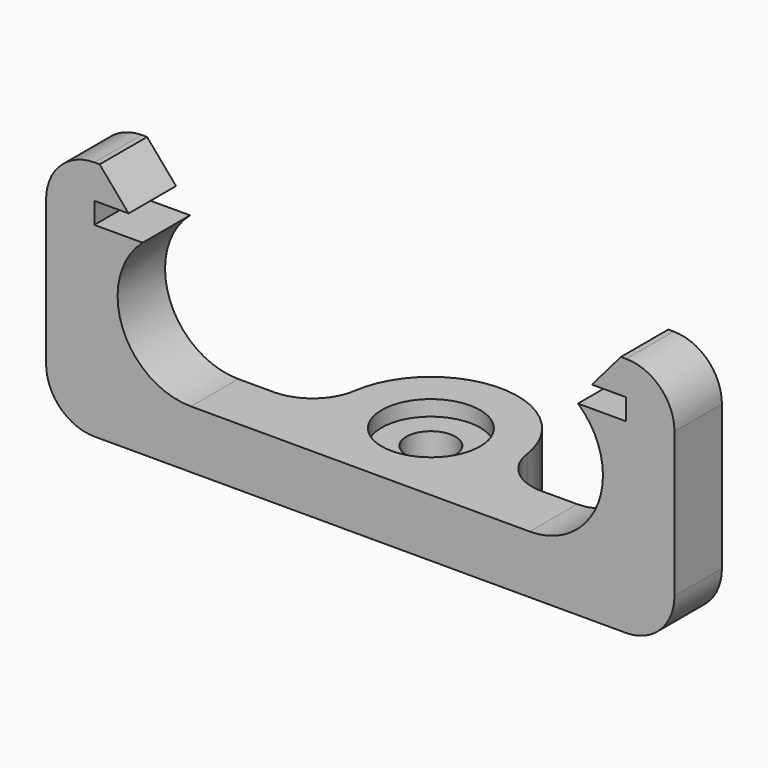
from build123d import *

# Parameters (mm, degrees)
F1_DEPTH = 6
F0_W     = 10
F0_H     = 6.1438416846
F2_DEPTH = 25
F3_DEPTH = 6
F0_R     = 2.55
F4_DEPTH = 4.4
F5_R     = 5
F7_DEPTH = 10


with BuildPart() as f1:
    # F0 (on Top) → F1 (new body)
    with BuildSketch(Plane.XY):
        with BuildLine():
            ThreePointArc((8.4852813742, -3), (0, -9), (-8.4852813742, -3))
            Line((-8.4852813742, -3), (-22.55, -3))
            Line((-22.55, -3), (-22.55, -9.1438416846))
            Line((-22.55, -9.1438416846), (22.55, -9.1438416846))
            Line((22.55, -9.1438416846), (22.55, -3))
            Line((22.55, -3), (8.4852813742, -3))
        make_face()
    extrude(amount=F1_DEPTH)

    # F0 (on Top) → F2 (join)
    with BuildSketch(Plane.XY):
        with Locations((-27.55, -6.0719208423)):
            Rectangle(F0_W, F0_H)
        with Locations((27.55, -6.0719208423)):
            Rectangle(F0_W, F0_H)
    extrude(amount=F2_DEPTH)

    # F0 (on Top) → F3 (join)
    with BuildSketch(Plane.XY):
        with BuildLine():
            ThreePointArc((-4.1243181255, -3), (-1.5773359756, 4.84994961), (5.1, 0))
            ThreePointArc((5.1, 0), (4.84994961, -1.5773359756), (4.1243181255, -3))
            Line((4.1243181255, -3), (8.4852813742, -3))
            ThreePointArc((8.4852813742, -3), (8.8703870369, -1.5219178085), (9, 0))
            ThreePointArc((9, 0), (-1.5219178085, 8.8703870369), (-8.4852813742, -3))
            Line((-8.4852813742, -3), (-4.1243181255, -3))
        make_face()
        with BuildLine():
            ThreePointArc((4.1243181255, -3), (0, -5.1), (-4.1243181255, -3))
            Line((-4.1243181255, -3), (-8.4852813742, -3))
            ThreePointArc((-8.4852813742, -3), (0, -9), (8.4852813742, -3))
            Line((8.4852813742, -3), (4.1243181255, -3))
        make_face()
    extrude(amount=F3_DEPTH)

    # F0 (on Top) → F4 (join)
    with BuildSketch(Plane.XY):
        with BuildLine():
            ThreePointArc((4.1243181255, -3), (4.84994961, -1.5773359756), (5.1, 0))
            ThreePointArc((5.1, 0), (-1.5773359756, 4.84994961), (-4.1243181255, -3))
            Line((-4.1243181255, -3), (4.1243181255, -3))
        make_face()
        Circle(F0_R, mode=Mode.SUBTRACT)
        with BuildLine():
            Line((4.1243181255, -3), (-4.1243181255, -3))
            ThreePointArc((-4.1243181255, -3), (0, -5.1), (4.1243181255, -3))
        make_face()
    extrude(amount=F4_DEPTH)

    # F5
    f5_edges = [f1.edges().sort_by_distance(p)[0] for p in [
        (-8.485281, -3, 3),
        (8.485281, -3, 3),
        (22.55, -6.071921, 6),
        (-22.55, -6.071921, 6),
        (-32.55, -6.071921, 0),
        (32.55, -6.071921, 0),
        (32.55, -6.071921, 25),
        (-32.55, -6.071921, 25),
    ]]
    fillet(f5_edges, radius=F5_R)

    # F6 (on face) → F7 (cut)
    with BuildSketch(Plane.XZ.offset(9.1438416846)):
        Polygon((17.55, 19.3), (22.55, 19.3), (22.55, 21.5), (-22.55, 21.5), (-22.55, 19.3), (-17.55, 19.3), align=None)
        Polygon((-22.55, 19.3), (-22.55, 21.5), (-24, 21.5), (-27.55, 21.5), (-27.55, 19.3), align=None)
        Polygon((22.55, 19.3), (27.55, 19.3), (27.55, 21.5), (24, 21.5), (22.55, 21.5), align=None)
        Polygon((-24, 21.5), (-22.55, 21.5), (-22.55, 25), (-27, 25), align=None)
        Polygon((22.55, 25), (22.55, 21.5), (24, 21.5), (27, 25), align=None)
        with BuildLine():
            ThreePointArc((-22.55, 19.3), (-24.654400045, 10.9190225395), (-17.55, 6))
            ThreePointArc((-17.55, 6), (-21.0855339059, 7.4644660941), (-22.55, 11))
            Line((-22.55, 11), (-22.55, 19.3))
        make_face()
        with BuildLine():
            ThreePointArc((17.55, 6), (24.654400045, 10.9190225395), (22.55, 19.3))
            Line((22.55, 19.3), (22.55, 11))
            ThreePointArc((22.55, 11), (21.0855339059, 7.4644660941), (17.55, 6))
        make_face()
    extrude(amount=-F7_DEPTH, mode=Mode.SUBTRACT)


solid = f1.part
